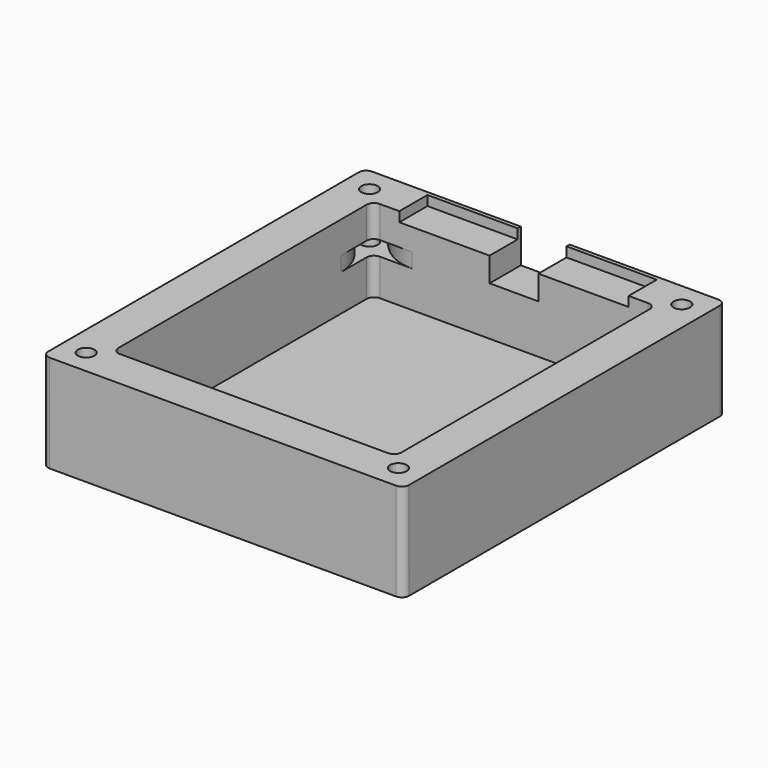
from build123d import *

# Parameters (mm, degrees)
F1_DEPTH  = 20
F2_DEPTH  = 3
F0_R      = 1.7
F3_DEPTH  = 10.5
F4_R      = 1.7
F5_DEPTH  = 6.5
F6_R      = 10
F7_R      = 1.5
F8_DEPTH  = 1.5
F9_W      = 10
F9_H      = 7
F10_DEPTH = 10
F12_W     = 18.5
F12_H     = 7.2
F13_DEPTH = 2


with BuildPart() as f1:
    # F0 (on Top) → F1 (new body)
    with BuildSketch(Plane.XY):
        Polygon((-37, 31.3), (-37, -41.3), (37, -41.3), (37, 31.3), (37, 41.3), (-37, 41.3), align=None)
        Polygon((-28.8793207629, 37.1391206695), (-25.0402000934, 33.3), (25.0402000934, 33.3), (28.8793207629, 37.1391206695), (31.1655111895, 39.4253110961), (34.2885053902, 38.5885073221), (35.1253091642, 35.4655131215), (32.8391187376, 33.1793226949), (29, 29.3402039573), (29, -29.3402039573), (32.8391187376, -33.1793226949), (35.1253091642, -35.4655131215), (34.2885053902, -38.5885073221), (31.1655111895, -39.4253110961), (28.8793207629, -37.1391206695), (25.0402000934, -33.3), (-25.0402000934, -33.3), (-28.8793207629, -37.1391206695), (-31.1655111895, -39.4253110961), (-34.2885053902, -38.5885073221), (-35.1253091642, -35.4655131215), (-32.8391187376, -33.1793226949), (-29, -29.3402039573), (-29, 29.3402039573), (-32.8391187376, 33.1793226949), (-35.1253091642, 35.4655131215), (-34.2885053902, 38.5885073221), (-31.1655111895, 39.4253110961), align=None, mode=Mode.SUBTRACT)
    extrude(amount=F1_DEPTH)

    # F0 (on Top) → F2 (join)
    with BuildSketch(Plane.XY):
        Polygon((-25.0402000934, 33.3), (-29, 33.3), (-29, 29.3402039573), (-29, -29.3402039573), (-29, -33.3), (-25.0402000934, -33.3), (25.0402000934, -33.3), (29, -33.3), (29, -29.3402039573), (29, 29.3402039573), (29, 33.3), (25.0402000934, 33.3), align=None)
    extrude(amount=F2_DEPTH)

    # F0 (on Top) → F3 (join)
    with BuildSketch(Plane.XY):
        Polygon((-29, 29.3402039573), (-29, 33.3), (-25.0402000934, 33.3), (-28.8793207629, 37.1391206695), (-29.716124537, 34.0161264689), (-32.8391187376, 33.1793226949), align=None)
        Polygon((-29.716124537, 34.0161264689), (-28.8793207629, 37.1391206695), (-31.1655111895, 39.4253110961), (-34.2885053902, 38.5885073221), (-35.1253091642, 35.4655131215), (-32.8391187376, 33.1793226949), align=None)
        with Locations((-32, 36.3)):
            Circle(F0_R, mode=Mode.SUBTRACT)
        Polygon((28.8793207629, 37.1391206695), (25.0402000934, 33.3), (29, 33.3), (29, 29.3402039573), (32.8391187376, 33.1793226949), (29.716124537, 34.0161264689), align=None)
        Polygon((31.1655111895, 39.4253110961), (28.8793207629, 37.1391206695), (29.716124537, 34.0161264689), (32.8391187376, 33.1793226949), (35.1253091642, 35.4655131215), (34.2885053902, 38.5885073221), align=None)
        with Locations((32, 36.3)):
            Circle(F0_R, mode=Mode.SUBTRACT)
        Polygon((32.8391187376, -33.1793226949), (29, -29.3402039573), (29, -33.3), (25.0402000934, -33.3), (28.8793207629, -37.1391206695), (29.716124537, -34.0161264689), align=None)
        Polygon((-29, -33.3), (-29, -29.3402039573), (-32.8391187376, -33.1793226949), (-29.716124537, -34.0161264689), (-28.8793207629, -37.1391206695), (-25.0402000934, -33.3), align=None)
        Polygon((-29.716124537, -34.0161264689), (-32.8391187376, -33.1793226949), (-35.1253091642, -35.4655131215), (-34.2885053902, -38.5885073221), (-31.1655111895, -39.4253110961), (-28.8793207629, -37.1391206695), align=None)
        with Locations((-32.0023149636, -36.3023168955)):
            Circle(F0_R, mode=Mode.SUBTRACT)
        Polygon((35.1253091642, -35.4655131215), (32.8391187376, -33.1793226949), (29.716124537, -34.0161264689), (28.8793207629, -37.1391206695), (31.1655111895, -39.4253110961), (34.2885053902, -38.5885073221), align=None)
        with Locations((32, -36.3)):
            Circle(F0_R, mode=Mode.SUBTRACT)
    extrude(amount=F3_DEPTH)

    # F4 (on face) → F5 (join)
    with BuildSketch(Plane.XY.offset(20)):
        Polygon((-29, -29.3402039573), (-32.8391187376, -33.1793226949), (-29.716124537, -34.0161264689), (-28.8793207629, -37.1391206695), (-25.0402000934, -33.3), (-29, -33.3), align=None)
        Polygon((-29.716124537, -34.0161264689), (-32.8391187376, -33.1793226949), (-35.1253091642, -35.4655131215), (-34.2885053902, -38.5885073221), (-31.1655111895, -39.4253110961), (-28.8793207629, -37.1391206695), align=None)
        with Locations((-32.0023149636, -36.3023168955)):
            Circle(F4_R, mode=Mode.SUBTRACT)
        Polygon((29, -33.3), (25.0402000934, -33.3), (28.8793207629, -37.1391206695), (29.716124537, -34.0161264689), (32.8391187376, -33.1793226949), (29, -29.3402039573), align=None)
        Polygon((29.716124537, -34.0161264689), (28.8793207629, -37.1391206695), (31.1655111895, -39.4253110961), (34.2885053902, -38.5885073221), (35.1253091642, -35.4655131215), (32.8391187376, -33.1793226949), align=None)
        with Locations((32, -36.3)):
            Circle(F4_R, mode=Mode.SUBTRACT)
        Polygon((28.8793207629, 37.1391206695), (25.0402000934, 33.3), (29, 33.3), (29, 29.3402039573), (32.8391187376, 33.1793226949), (29.716124537, 34.0161264689), align=None)
        Polygon((31.1655111895, 39.4253110961), (28.8793207629, 37.1391206695), (29.716124537, 34.0161264689), (32.8391187376, 33.1793226949), (35.1253091642, 35.4655131215), (34.2885053902, 38.5885073221), align=None)
        with Locations((32, 36.3)):
            Circle(F4_R, mode=Mode.SUBTRACT)
        Polygon((-32.8391187376, 33.1793226949), (-29, 29.3402039573), (-29, 33.3), (-25.0402000934, 33.3), (-28.8793207629, 37.1391206695), (-29.716124537, 34.0161264689), align=None)
        Polygon((-35.1253091642, 35.4655131215), (-32.8391187376, 33.1793226949), (-29.716124537, 34.0161264689), (-28.8793207629, 37.1391206695), (-31.1655111895, 39.4253110961), (-34.2885053902, 38.5885073221), align=None)
        with Locations((-32, 36.3)):
            Circle(F4_R, mode=Mode.SUBTRACT)
    extrude(amount=-F5_DEPTH)

    # F6
    f6_edges = [f1.edges().sort_by_distance(p)[0] for p in [
        (29, 29.340204, 12),
        (25.0402, 33.3, 12),
        (29, -29.340204, 12),
        (25.0402, -33.3, 12),
        (-29, 29.340204, 12),
        (-25.0402, 33.3, 12),
        (-25.0402, -33.3, 12),
        (-29, -29.340204, 12),
    ]]
    fillet(f6_edges, radius=F6_R)

    # F7
    f7_edges = [f1.edges().sort_by_distance(p)[0] for p in [
        (-37, -41.3, 10),
        (37, -41.3, 10),
        (-37, 41.3, 10),
        (37, 41.3, 10),
        (-29, 33.3, 6.75),
        (-29, 33.3, 16.75),
        (29, 33.3, 6.75),
        (29, 33.3, 16.75),
        (-29, -33.3, 6.75),
        (-29, -33.3, 16.75),
        (29, -33.3, 6.75),
        (29, -33.3, 16.75),
    ]]
    fillet(f7_edges, radius=F7_R)

    # F0 (on Top) → F8 (join)
    with BuildSketch(Plane.XY):
        with Locations((32, -36.3)):
            Circle(F0_R)
        with Locations((32, 36.3)):
            Circle(F0_R)
        with Locations((-32.0023149636, -36.3023168955)):
            Circle(F0_R)
        with Locations((-32, 36.3)):
            Circle(F0_R)
    extrude(amount=F8_DEPTH)

    # F9 (on face) → F10 (cut)
    with BuildSketch(Plane(origin=(0, 41.3, 0), x_dir=(-1, 0, 0), z_dir=(0, 1, 0))):
        with Locations((0, 16.5)):
            Rectangle(F9_W, F9_H)
    extrude(amount=-F10_DEPTH, mode=Mode.SUBTRACT)

    # F12 (on face) → F13 (cut)
    with BuildSketch(Plane.XY.offset(20)):
        with Locations((-14.25, 36.9)):
            Rectangle(F12_W, F12_H)
        with Locations((14.25, 36.9)):
            Rectangle(F12_W, F12_H)
    extrude(amount=-F13_DEPTH, mode=Mode.SUBTRACT)


solid = f1.part
